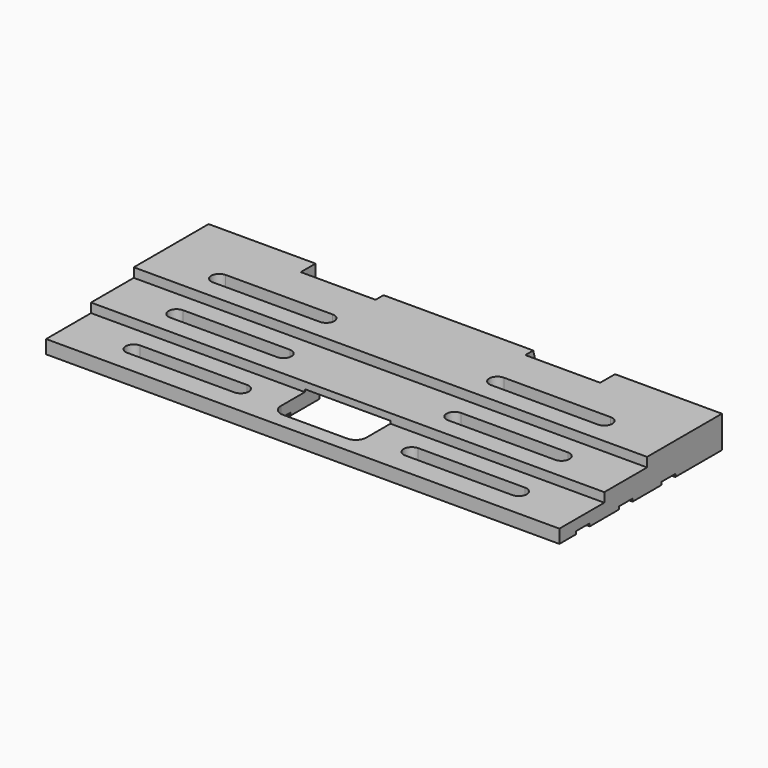
from build123d import *

# Parameters (mm, degrees)
F0_W         = 609.6
F0_H         = 241.3
F1_DEPTH     = 38.1
F3_DEPTH     = 38.101
F4_W         = 76.2
F4_H         = 50.8
F5_DEPTH     = 19.05
F6_R         = 12.7
F8_DEPTH     = 88.9
F10_DEPTH    = 88.9
F11_W        = 609.6
F11_H        = 66.675
F12_DEPTH    = 22.098
F13_W        = 609.6
F13_H        = 63.5
F14_DEPTH    = 11.049
F15_W        = 101.6
F15_H        = 191.5146559477
F16_DEPTH    = 19.05
F17_T1_DEPTH = 19.05
F17_T3_DEPTH = 16.002
F18_W        = 20.32
F18_H        = 3.302
F19_DEPTH    = 609.601


# Not quite as in the source:
# - a fillet or chamfer that OpenCascade refuses, or shapes differently, is made with other operations: its cross-section is extruded or revolved along the edge and cut away or added
# - a pattern or mirror of a feature is missing from the dataset's text; its kind, count and spacing are read off the source's solid


with BuildPart() as f1:
    # F0 (on Top) → F1 (new body)
    with BuildSketch(Plane.XY):
        Rectangle(F0_W, F0_H)
    extrude(amount=F1_DEPTH)

    # F2 (on face) → F3 (cut, through all)
    with BuildSketch(Plane.XY.offset(38.1)):
        with BuildLine():
            Line((-101.6, -76.2), (-228.6, -76.2))
            ThreePointArc((-228.6, -76.2), (-238.125, -85.725), (-228.6, -95.25))
            Line((-228.6, -95.25), (-101.6, -95.25))
            ThreePointArc((-101.6, -95.25), (-92.075, -85.725), (-101.6, -76.2))
        make_face()
        with BuildLine():
            Line((-228.6, -31.75), (-101.6, -31.75))
            ThreePointArc((-101.6, -31.75), (-92.075, -22.225), (-101.6, -12.7))
            Line((-101.6, -12.7), (-228.6, -12.7))
            ThreePointArc((-228.6, -12.7), (-238.125, -22.225), (-228.6, -31.75))
        make_face()
        with BuildLine():
            Line((-228.6, 31.75), (-101.6, 31.75))
            ThreePointArc((-101.6, 31.75), (-92.075, 41.275), (-101.6, 50.8))
            Line((-101.6, 50.8), (-228.6, 50.8))
            ThreePointArc((-228.6, 50.8), (-238.125, 41.275), (-228.6, 31.75))
        make_face()
    f3 = extrude(amount=-F3_DEPTH, mode=Mode.SUBTRACT)

    # F3_copies: F3 across plane
    add(f3.mirror(Plane(origin=(0, 0, 0), x_dir=(0, 0, 1), z_dir=(1, 0, 0))), mode=Mode.SUBTRACT)

    # F4 (on face) → F5 (cut)
    with BuildSketch(Plane(origin=(0, 0, 0), x_dir=(1, 0, 0), z_dir=(0, 0, -1))):
        with Locations((241.3, -95.25)):
            Rectangle(F4_W, F4_H)
    f5 = extrude(amount=-F5_DEPTH, mode=Mode.SUBTRACT)

    # F5_copies: F5 across plane
    add(f5.mirror(Plane(origin=(0, 0, 0), x_dir=(0, 0, -1), z_dir=(-1, 0, 0))), mode=Mode.SUBTRACT)

    # F6
    f6_edges = [f1.edges().sort_by_distance(p)[0] for p in [
        (279.4, 69.85, 9.525),
        (203.2, 69.85, 9.525),
    ]]
    fillet(f6_edges, radius=F6_R)

    # F7 (on Right) → F8 (cut, symmetric)
    with BuildSketch(Plane.YZ):
        Polygon((120.65, 38.1), (110.4411357684, 38.1), (120.65, 0), align=None)
    extrude(amount=F8_DEPTH, both=True, mode=Mode.SUBTRACT)

    # F9 (on face) → F10 (cut)
    with BuildSketch(Plane.YZ.offset(-88.9)):
        Polygon((98.6529547439, 38.1), (120.65, 0), (120.65, 38.1), align=None)
    f10 = extrude(amount=-F10_DEPTH, mode=Mode.SUBTRACT)

    # F10_copies: F10 across plane
    add(f10.mirror(Plane(origin=(0, 0, 0), x_dir=(0, 0, 1), z_dir=(1, 0, 0))), mode=Mode.SUBTRACT)

    # F11 (on face) → F12 (cut)
    with BuildSketch(Plane.XY.offset(38.1)):
        with Locations((0, -87.3125)):
            Rectangle(F11_W, F11_H)
    extrude(amount=-F12_DEPTH, mode=Mode.SUBTRACT)

    # F13 (on face) → F14 (cut)
    with BuildSketch(Plane.XY.offset(38.1)):
        with Locations((0, -22.225)):
            Rectangle(F13_W, F13_H)
    extrude(amount=-F14_DEPTH, mode=Mode.SUBTRACT)

    # F15 (on face) → F16 (cut)
    with BuildSketch(Plane(origin=(0, 0, 0), x_dir=(1, 0, 0), z_dir=(0, 0, -1))):
        with Locations((0, 6.5381005406)):
            Rectangle(F15_W, F15_H)
    extrude(amount=-F16_DEPTH, mode=Mode.SUBTRACT)

    # F17: fillet of radius 12.7 on 6 edges, made by hand

    # F17_s2 → F17_t1 (join)
    with BuildSketch(Plane.XY):
        with BuildLine():
            ThreePointArc((-50.8004, 76.5182617478), (-47.0802561211, 85.4994835543), (-38.0990343146, 89.2196274332))
            Line((-38.0990343146, 89.2196274332), (-38.0990343146, 90.4897640017))
            ThreePointArc((-38.0990343146, 90.4897640017), (-44.4495171573, 90.4893640017), (-50.8, 90.4893640017))
            Line((-50.8, 90.4893640017), (-52.0701365685, 89.2192274332))
            ThreePointArc((-52.0701365685, 89.2192274332), (-52.0701365685, 82.8687445905), (-52.0705365685, 76.5182617478))
            Line((-52.0705365685, 76.5182617478), (-50.8004, 76.5182617478))
        make_face()
        with BuildLine():
            ThreePointArc((50.8004, 76.5182617478), (47.0802561211, 85.4994835543), (38.0990343146, 89.2196274332))
            Line((38.0990343146, 89.2196274332), (38.0990343146, 90.4897640017))
            ThreePointArc((38.0990343146, 90.4897640017), (44.4495171573, 90.4893640017), (50.8, 90.4893640017))
            Line((50.8, 90.4893640017), (52.0701365685, 89.2192274332))
            ThreePointArc((52.0701365685, 89.2192274332), (52.0701365685, 82.8687445905), (52.0705365685, 76.5182617478))
            Line((52.0705365685, 76.5182617478), (50.8004, 76.5182617478))
        make_face()
        with BuildLine():
            ThreePointArc((-203.1996, 82.5509656854), (-206.9197438789, 73.5697438789), (-215.9009656854, 69.8496))
            Line((-215.9009656854, 69.8496), (-215.9009656854, 68.5794634315))
            ThreePointArc((-215.9009656854, 68.5794634315), (-209.5504828427, 68.5798634315), (-203.2, 68.5798634315))
            Line((-203.2, 68.5798634315), (-201.9298634315, 69.85))
            ThreePointArc((-201.9298634315, 69.85), (-201.9298634315, 76.2004828427), (-201.9294634315, 82.5509656854))
            Line((-201.9294634315, 82.5509656854), (-203.1996, 82.5509656854))
        make_face()
        with BuildLine():
            ThreePointArc((-266.6990343146, 69.8496), (-275.6802561211, 73.5697438789), (-279.4004, 82.5509656854))
            Line((-279.4004, 82.5509656854), (-280.6705365685, 82.5509656854))
            ThreePointArc((-280.6705365685, 82.5509656854), (-280.6701365685, 76.2004828427), (-280.6701365685, 69.85))
            Line((-280.6701365685, 69.85), (-279.4, 68.5798634315))
            ThreePointArc((-279.4, 68.5798634315), (-273.0495171573, 68.5798634315), (-266.6990343146, 68.5794634315))
            Line((-266.6990343146, 68.5794634315), (-266.6990343146, 69.8496))
        make_face()
    extrude(amount=F17_T1_DEPTH)

    # F17_s4 → F17_t3 (join)
    with BuildSketch(Plane.XY):
        with BuildLine():
            ThreePointArc((-50.8004, -89.5944628291), (-47.0802561211, -98.5756846355), (-38.0990343146, -102.2958285145))
            Line((-38.0990343146, -102.2958285145), (-38.0990343146, -103.565965083))
            ThreePointArc((-38.0990343146, -103.565965083), (-44.4495171573, -103.565565083), (-50.8, -103.565565083))
            Line((-50.8, -103.565565083), (-52.0701365685, -102.2954285145))
            ThreePointArc((-52.0701365685, -102.2954285145), (-52.0701365685, -95.9449456718), (-52.0705365685, -89.5944628291))
            Line((-52.0705365685, -89.5944628291), (-50.8004, -89.5944628291))
        make_face()
        with BuildLine():
            ThreePointArc((38.0990343146, -102.2958285145), (47.0802561211, -98.5756846355), (50.8004, -89.5944628291))
            Line((50.8004, -89.5944628291), (52.0705365685, -89.5944628291))
            ThreePointArc((52.0705365685, -89.5944628291), (52.0701365685, -95.9449456718), (52.0701365685, -102.2954285145))
            Line((52.0701365685, -102.2954285145), (50.8, -103.565565083))
            ThreePointArc((50.8, -103.565565083), (44.4495171573, -103.565565083), (38.0990343146, -103.565965083))
            Line((38.0990343146, -103.565965083), (38.0990343146, -102.2958285145))
        make_face()
    extrude(amount=F17_T3_DEPTH)

    # F18 (on face) → F19 (cut, through all)
    with BuildSketch(Plane(origin=(-304.8, 0, 0), x_dir=(0, -1, 0), z_dir=(-1, 0, 0))):
        with Locations((-41.275, 1.651)):
            Rectangle(F18_W, F18_H)
        with Locations((22.225, 1.651)):
            Rectangle(F18_W, F18_H)
        with Locations((85.725, 1.651)):
            Rectangle(F18_W, F18_H)
    extrude(amount=-F19_DEPTH, mode=Mode.SUBTRACT)


solid = f1.part
